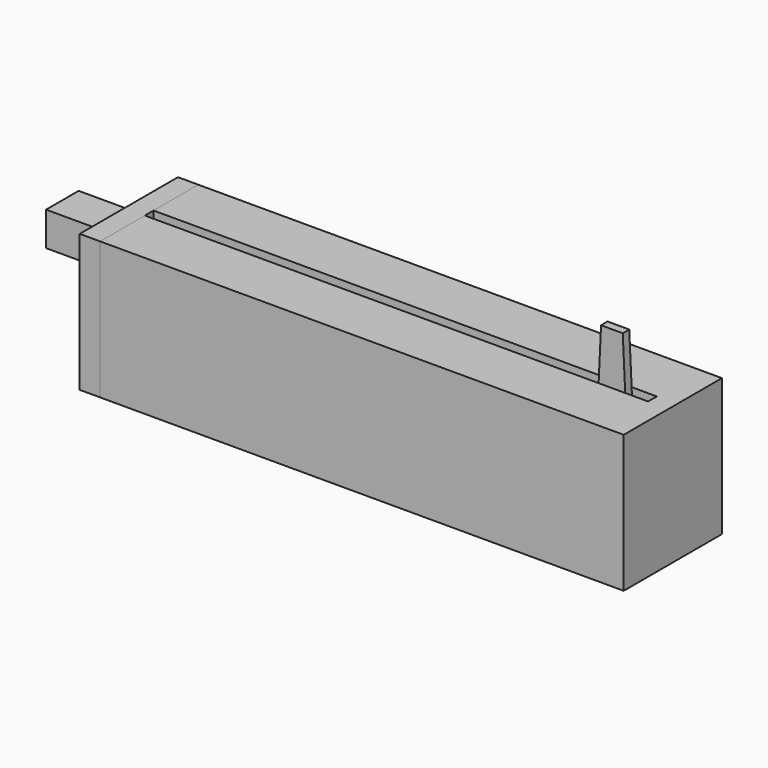
from build123d import *

# Parameters (mm, degrees)
F0_W      = 74.2
F0_H      = 9.3
F1_DEPTH  = 6.35
F2_W      = 67.2
F2_H      = 2.7
F3_DEPTH  = 5
F7_DEPTH  = 0.6
F9_W      = 87
F9_H      = 6
F9_W_2    = 5
F9_H_2    = 1.2
F10_DEPTH = 5
F13_DEPTH = 74.2
F14_W     = 18.1
F14_H     = 20.25
F15_DEPTH = 3
F18_W     = 4
F18_H     = 7
F19_DEPTH = 10
F21_DEPTH = 10
F23_DEPTH = 20
F17_W     = 18.1
F17_H     = 20.25
F24_DEPTH = 3
F25_DEPTH = 3


with BuildPart() as f1:
    # F0 (on Top) → F1 (new body)
    with BuildSketch(Plane.XY):
        with Locations((-0.6390025849, -4.65)):
            Rectangle(F0_W, F0_H)
    extrude(amount=F1_DEPTH)

    # F2 (on face) → F3 (cut)
    with BuildSketch(Plane.XY.offset(6.35)):
        with Locations((-0.1390025849, -4.65)):
            Rectangle(F2_W, F2_H)
    extrude(amount=-F3_DEPTH, mode=Mode.SUBTRACT)


with BuildPart() as f1_1:
    # F5: moved
    add(f1.part.moved(Location((0, 4.65, 0))))


with BuildPart() as f7:
    # F6 (on Front) → F7 (new body, symmetric)
    with BuildSketch(Plane.XZ):
        Polygon((28.4609974151, 11.35), (28.4609974151, 0.2899478026), (33.4609974151, 0.2899478026), (33.4609974151, 11.35), (32.5359974151, 11.35), (32.5359974151, 12.3243909329), (32.9609974151, 12.85), (32.5609974151, 21.35), (30.9609974151, 21.35), (29.3609974151, 21.35), (28.9609974151, 12.85), (29.3859974151, 12.3243909329), (29.3859974151, 11.35), align=None)
    extrude(amount=F7_DEPTH, both=True)


with BuildPart() as f10:
    # F9 (on offset) → F10 (new body)
    with BuildSketch(Plane.XY.offset(6.35)):
        with Locations((-7.0390025849, 0)):
            Rectangle(F9_W, F9_H)
        with Locations((30.9609974151, 0)):
            Rectangle(F9_W_2, F9_H_2, mode=Mode.SUBTRACT)
    extrude(amount=F10_DEPTH)

    # F20 (on face) → F21 (cut)
    with BuildSketch(Plane(origin=(-50.5390025849, 0, 0), x_dir=(0, -1, 0), z_dir=(-1, 0, 0))):
        with BuildLine():
            ThreePointArc((1.375, 8.85), (0.9722718241, 9.8222718241), (0, 10.225))
            Line((0, 10.225), (0, 7.475))
            ThreePointArc((0, 7.475), (0.9722718241, 7.8777281759), (1.375, 8.85))
        make_face()
        with BuildLine():
            Line((0, 7.475), (0, 10.225))
            ThreePointArc((0, 10.225), (-1.375, 8.85), (0, 7.475))
        make_face()
    extrude(amount=-F21_DEPTH, mode=Mode.SUBTRACT)


with BuildPart() as f13:
    # F12 (on offset) → F13 (new body)
    with BuildSketch(Plane.YZ.offset(36.4609974151)):
        Polygon((-9.05, 13.85), (-9.05, -6.4), (0, -6.4), (0, -4.4), (-2.45, -4.4), (-2.45, -0.4), (-5.05, -0.4), (-5.05, 6.75), (-3.4, 6.75), (-3.4, 11.85), (-0.8, 11.85), (-0.8, 13.85), align=None)
        Polygon((0, -4.4), (0, -6.4), (9.05, -6.4), (9.05, 13.85), (0.8, 13.85), (0.8, 11.85), (3.4, 11.85), (3.4, 6.75), (5.05, 6.75), (5.05, -0.4), (2.45, -0.4), (2.45, -4.4), align=None)
    extrude(amount=-F13_DEPTH)

    # F14 (on offset) → F15 (join)
    with BuildSketch(Plane.YZ.offset(36.4609974151)):
        with Locations((0, 3.725)):
            Rectangle(F14_W, F14_H)
    extrude(amount=F15_DEPTH)

    # F18 (on face) → F19 (cut)
    with BuildSketch(Plane(origin=(0, 0, -6.4), x_dir=(1, 0, 0), z_dir=(0, 0, -1))):
        with Locations((-35.7390025849, 0)):
            Rectangle(F18_W, F18_H)
        with Locations((34.4609974151, 0)):
            Rectangle(F18_W, F18_H)
    extrude(amount=-F19_DEPTH, mode=Mode.SUBTRACT)

    # F22 (on face) → F23 (cut)
    with BuildSketch(Plane(origin=(-37.7390025849, 0, 0), x_dir=(0, -1, 0), z_dir=(-1, 0, 0))):
        with BuildLine():
            Line((-6.225, 10.3), (-4.725, 10.3))
            ThreePointArc((-4.725, 10.3), (-5.1643398282, 11.3606601718), (-6.225, 11.8))
            Line((-6.225, 11.8), (-6.225, 10.3))
        make_face()
        with BuildLine():
            ThreePointArc((-6.225, 8.8), (-5.1643398282, 9.2393398282), (-4.725, 10.3))
            Line((-4.725, 10.3), (-6.225, 10.3))
            Line((-6.225, 10.3), (-6.225, 8.8))
        make_face()
        with BuildLine():
            Line((-6.225, 10.3), (-6.225, 11.8))
            ThreePointArc((-6.225, 11.8), (-7.2856601718, 11.3606601718), (-7.725, 10.3))
            Line((-7.725, 10.3), (-6.225, 10.3))
        make_face()
        with BuildLine():
            ThreePointArc((-7.725, 10.3), (-7.2856601718, 9.2393398282), (-6.225, 8.8))
            Line((-6.225, 8.8), (-6.225, 10.3))
            Line((-6.225, 10.3), (-7.725, 10.3))
        make_face()
        with BuildLine():
            Line((6.275, -3.4), (7.775, -3.4))
            ThreePointArc((7.775, -3.4), (7.3356601718, -2.3393398282), (6.275, -1.9))
            Line((6.275, -1.9), (6.275, -3.4))
        make_face()
        with BuildLine():
            ThreePointArc((6.275, -4.9), (7.3356601718, -4.4606601718), (7.775, -3.4))
            Line((7.775, -3.4), (6.275, -3.4))
            Line((6.275, -3.4), (6.275, -4.9))
        make_face()
        with BuildLine():
            Line((6.275, -3.4), (6.275, -1.9))
            ThreePointArc((6.275, -1.9), (5.2143398282, -2.3393398282), (4.775, -3.4))
            Line((4.775, -3.4), (6.275, -3.4))
        make_face()
        with BuildLine():
            ThreePointArc((4.775, -3.4), (5.2143398282, -4.4606601718), (6.275, -4.9))
            Line((6.275, -4.9), (6.275, -3.4))
            Line((6.275, -3.4), (4.775, -3.4))
        make_face()
    extrude(amount=-F23_DEPTH, mode=Mode.SUBTRACT)


with BuildPart() as f24:
    # F17 (on offset) → F24 (new body)
    with BuildSketch(Plane(origin=(-37.7390025849, 0, 0), x_dir=(0, -1, 0), z_dir=(-1, 0, 0))):
        with Locations((0, 3.725)):
            Rectangle(F17_W, F17_H)
        Polygon((-3.4, 6.75), (-3.4, 11.85), (3.4, 11.85), (3.4, 5.95), (-3.4, 5.95), (-3.4, 6.35), align=None, mode=Mode.SUBTRACT)
    extrude(amount=F24_DEPTH)

    # F22 (on face) → F25 (cut, through all)
    with BuildSketch(Plane(origin=(-37.7390025849, 0, 0), x_dir=(0, -1, 0), z_dir=(-1, 0, 0))):
        with BuildLine():
            Line((-6.225, 10.3), (-4.725, 10.3))
            ThreePointArc((-4.725, 10.3), (-5.1643398282, 11.3606601718), (-6.225, 11.8))
            Line((-6.225, 11.8), (-6.225, 10.3))
        make_face()
        with BuildLine():
            ThreePointArc((-6.225, 8.8), (-5.1643398282, 9.2393398282), (-4.725, 10.3))
            Line((-4.725, 10.3), (-6.225, 10.3))
            Line((-6.225, 10.3), (-6.225, 8.8))
        make_face()
        with BuildLine():
            Line((-6.225, 10.3), (-6.225, 11.8))
            ThreePointArc((-6.225, 11.8), (-7.2856601718, 11.3606601718), (-7.725, 10.3))
            Line((-7.725, 10.3), (-6.225, 10.3))
        make_face()
        with BuildLine():
            ThreePointArc((-7.725, 10.3), (-7.2856601718, 9.2393398282), (-6.225, 8.8))
            Line((-6.225, 8.8), (-6.225, 10.3))
            Line((-6.225, 10.3), (-7.725, 10.3))
        make_face()
        with BuildLine():
            Line((6.275, -3.4), (7.775, -3.4))
            ThreePointArc((7.775, -3.4), (7.3356601718, -2.3393398282), (6.275, -1.9))
            Line((6.275, -1.9), (6.275, -3.4))
        make_face()
        with BuildLine():
            ThreePointArc((6.275, -4.9), (7.3356601718, -4.4606601718), (7.775, -3.4))
            Line((7.775, -3.4), (6.275, -3.4))
            Line((6.275, -3.4), (6.275, -4.9))
        make_face()
        with BuildLine():
            Line((6.275, -3.4), (6.275, -1.9))
            ThreePointArc((6.275, -1.9), (5.2143398282, -2.3393398282), (4.775, -3.4))
            Line((4.775, -3.4), (6.275, -3.4))
        make_face()
        with BuildLine():
            ThreePointArc((4.775, -3.4), (5.2143398282, -4.4606601718), (6.275, -4.9))
            Line((6.275, -4.9), (6.275, -3.4))
            Line((6.275, -3.4), (4.775, -3.4))
        make_face()
    extrude(amount=F25_DEPTH, mode=Mode.SUBTRACT)


solid = Compound([f1_1.part, f7.part, f10.part, f13.part, f24.part])
